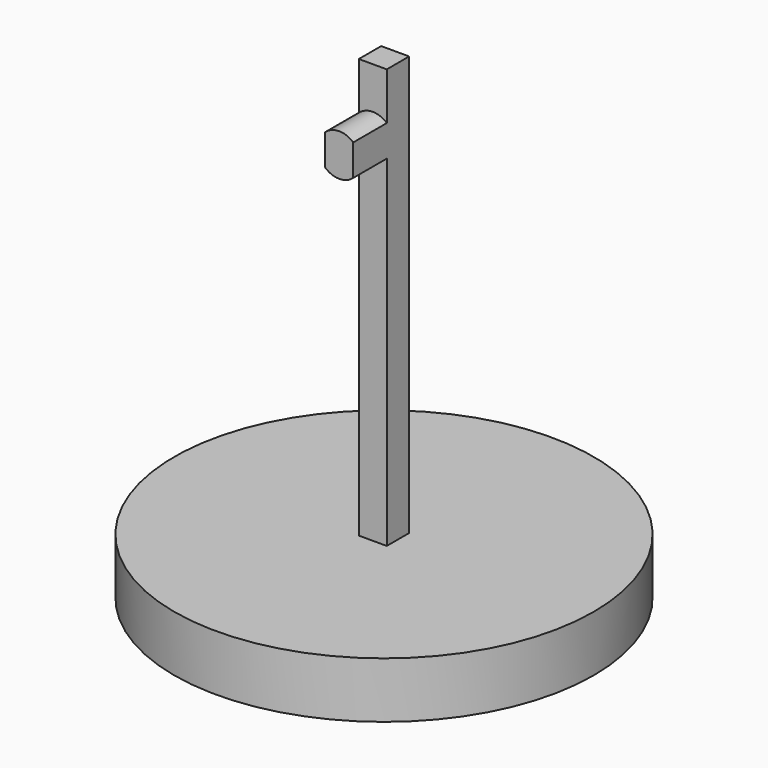
from build123d import *

# Parameters (mm, degrees)
F0_R     = 75
F1_DEPTH = 20
F2_W     = 10
F2_H     = 10
F3_DEPTH = 150
F5_DEPTH = 15


with BuildPart() as f1:
    # F0 (on Top) → F1 (new body)
    with BuildSketch(Plane.XY):
        Circle(F0_R)
    extrude(amount=F1_DEPTH)


with BuildPart() as f3:
    # F2 (on face) → F3 (new body)
    with BuildSketch(Plane.XY.offset(20)):
        Rectangle(F2_W, F2_H)
    extrude(amount=F3_DEPTH)

    # F4 (on face) → F5 (join)
    with BuildSketch(Plane.XZ.offset(5)):
        with BuildLine():
            Line((5, 141.9098300563), (5, 153.0901699437))
            ThreePointArc((5, 153.0901699437), (0, 155), (-5, 153.0901699437))
            Line((-5, 153.0901699437), (-5, 141.9098300563))
            ThreePointArc((-5, 141.9098300563), (0, 140), (5, 141.9098300563))
        make_face()
    extrude(amount=F5_DEPTH)


solid = Compound([f1.part, f3.part])
